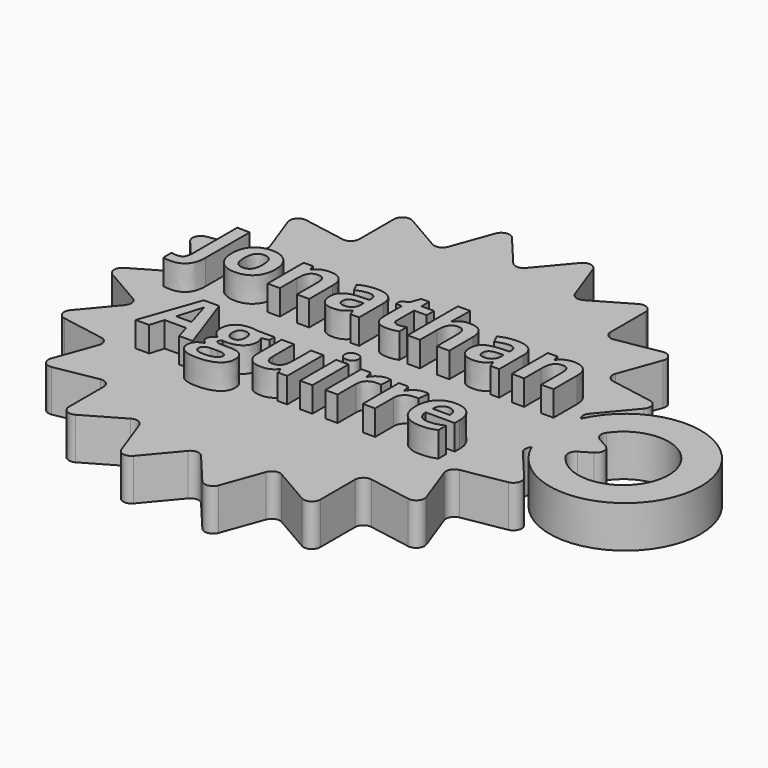
from build123d import *

# Parameters (mm, degrees)
F1_DEPTH      = 5
F2_R          = 1
F3_R          = 1
F4_R          = 9.02426598
F5_DEPTH      = 5
F7_DEPTH      = 5
F8_R          = 1
F10_DEPTH     = 4.5
F11_R         = 7.0893465871
F11_R_2       = 5.3736476411
F12_DEPTH     = 4.5
F13_TEXT_SIZE = 9.8616627859
F14_DEPTH     = 3


# Not quite as in the source:
# - a feature names something its author has since deleted; it is built from what else it names
# - Text() gives the source's letters only with a copy of the font that has no kerning and outlines rounded to 1/6400 em; it was checked with that copy


with BuildPart() as f1:
    # F0 (on Top) → F1 (new body)
    with BuildSketch(Plane.XY):
        Polygon((-69.4327632519, 10.2606042998), (-64.2233179219, 4.0522291123), (-71.2419846284, 0), (-64.2233179219, -4.0522291123), (-69.4327632519, -10.2606042998), (-61.4514299584, -11.6679287015), (-64.2233179219, -19.2836282906), (-56.2419846284, -17.8763038889), (-56.2419846284, -25.9807621135), (-49.2233179219, -21.9285330012), (-46.4514299584, -29.5442325904), (-41.2419846284, -23.3358574029), (-36.0325392983, -29.5442325904), (-33.2606513348, -21.9285330012), (-26.2419846284, -25.9807621135), (-26.2419846284, -17.8763038889), (-18.2606513348, -19.2836282906), (-21.0325392984, -11.6679287015), (-13.0512060048, -10.2606042998), (-18.2606513348, -4.0522291123), (-11.2419846284, 0), (-18.2606513348, 4.0522291123), (-13.0512060048, 10.2606042998), (-21.0325392984, 11.6679287015), (-18.2606513348, 19.2836282906), (-26.2419846284, 17.8763038889), (-26.2419846284, 25.9807621135), (-33.2606513348, 21.9285330012), (-36.0325392984, 29.5442325904), (-41.2419846284, 23.3358574029), (-46.4514299584, 29.5442325904), (-49.2233179219, 21.9285330012), (-56.2419846284, 25.9807621135), (-56.2419846284, 17.8763038889), (-64.2233179219, 19.2836282906), (-61.4514299584, 11.6679287015), align=None)
    extrude(amount=F1_DEPTH)

    # F2
    f2_edges = [f1.edges().sort_by_distance(p)[0] for p in [
        (-49.223318, -21.928533, 2.5),
        (-56.241985, -17.876304, 2.5),
        (-61.45143, -11.667929, 2.5),
        (-64.223318, -4.052229, 2.5),
        (-64.223318, 4.052229, 2.5),
        (-61.45143, 11.667929, 2.5),
        (-56.241985, 17.876304, 2.5),
        (-49.223318, 21.928533, 2.5),
        (-41.241985, 23.335857, 2.5),
        (-33.260651, 21.928533, 2.5),
        (-41.241985, -23.335857, 2.5),
        (-33.260651, -21.928533, 2.5),
        (-26.241985, -17.876304, 2.5),
        (-21.032539, -11.667929, 2.5),
        (-26.241985, 17.876304, 2.5),
        (-21.032539, 11.667929, 2.5),
        (-18.260651, 4.052229, 2.5),
        (-18.260651, -4.052229, 2.5),
    ]]
    fillet(f2_edges, radius=F2_R)

    # F3
    f3_edges = [f1.edges().sort_by_distance(p)[0] for p in [
        (-36.032539, 29.544233, 2.5),
        (-26.241985, 25.980762, 2.5),
        (-18.260651, 19.283628, 2.5),
        (-13.051206, 10.260604, 2.5),
        (-11.241985, 0, 2.5),
        (-13.051206, -10.260604, 2.5),
        (-56.241985, 25.980762, 2.5),
        (-46.45143, 29.544233, 2.5),
        (-64.223318, 19.283628, 2.5),
        (-69.432763, 10.260604, 2.5),
        (-71.241985, 0, 2.5),
        (-69.432763, -10.260604, 2.5),
        (-64.223318, -19.283628, 2.5),
        (-56.241985, -25.980762, 2.5),
        (-46.45143, -29.544233, 2.5),
        (-36.032539, -29.544233, 2.5),
        (-26.241985, -25.980762, 2.5),
        (-18.260651, -19.283628, 2.5),
    ]]
    fillet(f3_edges, radius=F3_R)

    # F4 (on Top) → F5 (join, through all)
    with BuildSketch(Plane.XY):
        with Locations((-9.2419846284, 0)):
            Circle(F4_R)
    extrude(amount=F5_DEPTH)

    # F6 (on face) → F7 (cut, through all)
    with BuildSketch(Plane.XY.offset(5)):
        with BuildLine():
            ThreePointArc((-14.3705448136, -2.1852792706), (-3.981082649, -0.0942598595), (-14.3705448136, 1.9967595517))
            Line((-14.3705448136, 1.9967595517), (-10.7515631244, 0))
            Line((-10.7515631244, 0), (-14.3705448136, -2.1852792706))
        make_face()
    extrude(amount=-F7_DEPTH, mode=Mode.SUBTRACT)

    # F8
    f8_edges = [f1.edges().sort_by_distance(p)[0] for p in [
        (-10.751563, 0, 2.5),
        (-14.370545, -2.185279, 2.5),
        (-14.370545, 1.99676, 2.5),
    ]]
    fillet(f8_edges, radius=F8_R)

    # F9 (on face) → F10 (cut)
    with BuildSketch(Plane.XY):
        with BuildLine():
            ThreePointArc((-35.3777156799, -4.6599307489), (-35.5753046169, -4.908160303), (-35.7829730175, -5.1480209603))
            Line((-35.7829730175, -5.1480209603), (-21.9766725259, -17.609254409))
            Line((-21.9766725259, -17.609254409), (-20.5904544794, -15.9396992978))
            Line((-20.5904544794, -15.9396992978), (-35.3777156799, -4.6599307489))
        make_face()
        with BuildLine():
            Line((-35.0430152336, -4.1849240607), (-22.1269458204, -12.5734481191))
            Line((-22.1269458204, -12.5734481191), (-20.8090839907, -10.2629405882))
            Line((-20.8090839907, -10.2629405882), (-34.6043804511, -3.4158988524))
            ThreePointArc((-34.6043804511, -3.4158988524), (-34.8126121734, -3.8067344742), (-35.0430152336, -4.1849240607))
        make_face()
        with BuildLine():
            ThreePointArc((-34.1823081919, -2.3833949122), (-34.2698744439, -2.6366901562), (-34.3662212872, -2.8867773708))
            Line((-34.3662212872, -2.8867773708), (-17.1305497448, -9.8744736155))
            Line((-17.1305497448, -9.8744736155), (-16.3989523541, -7.8314905025))
            Line((-16.3989523541, -7.8314905025), (-19.4509472573, -6.8787666419))
            Line((-19.4509472573, -6.8787666419), (-34.1823081919, -2.3833949122))
        make_face()
        with BuildLine():
            Line((-34.0002869576, -1.7286818538), (-18.9941076397, -5.1937600989))
            Line((-18.9941076397, -5.1937600989), (-18.54596272, -2.5718579299))
            Line((-18.54596272, -2.5718579299), (-33.8511272013, -0.8560126092))
            ThreePointArc((-33.8511272013, -0.8560126092), (-33.9131273587, -1.2944974025), (-34.0002869576, -1.7286818538))
        make_face()
        with BuildLine():
            ThreePointArc((-33.8115942061, 0.3570473634), (-33.8033972316, 0.0398847724), (-33.8083009973, -0.2773458261))
            Line((-33.8083009973, -0.2773458261), (-15.2221347635, -0.9486855723))
            Line((-15.2221347635, -0.9486855723), (-15.2333994712, 1.2213116278))
            Line((-15.2333994712, 1.2213116278), (-33.8115942061, 0.3570473634))
        make_face()
        with BuildLine():
            Line((-33.8605272028, 0.9360648973), (-18.5742046736, 2.812372041))
            Line((-18.5742046736, 2.812372041), (-19.0498295551, 5.4294287513))
            Line((-19.0498295551, 5.4294287513), (-34.0188333405, 1.807121388))
            ThreePointArc((-34.0188333405, 1.807121388), (-33.9271237992, 1.3738751607), (-33.8605272028, 0.9360648973))
        make_face()
        with BuildLine():
            ThreePointArc((-34.3965754224, 2.9605459736), (-34.2803967911, 2.6653141576), (-34.1765055688, 2.3655377184))
            Line((-34.1765055688, 2.3655377184), (-16.481610594, 8.0915279521))
            Line((-16.481610594, 8.0915279521), (-17.2343787101, 10.1268055511))
            Line((-17.2343787101, 10.1268055511), (-34.3965754224, 2.9605459736))
        make_face()
        with BuildLine():
            Line((-34.6405930582, 3.4879084069), (-20.9178834168, 10.4792906065))
            Line((-20.9178834168, 10.4792906065), (-22.2599107194, 12.7758461952))
            Line((-22.2599107194, 12.7758461952), (-35.0872710335, 4.2522898756))
            ThreePointArc((-35.0872710335, 4.2522898756), (-34.8529133175, 3.8765381033), (-34.6405930582, 3.4879084069))
        make_face()
        with BuildLine():
            ThreePointArc((-35.8367269225, 5.2069590463), (-35.6265794919, 4.9692673195), (-35.4264240963, 4.7231025025))
            Line((-35.4264240963, 4.7231025025), (-20.7570658633, 16.1557837872))
            Line((-20.7570658633, 16.1557837872), (-22.1605424433, 17.8108572693))
            Line((-22.1605424433, 17.8108572693), (-35.8367269225, 5.2069590463))
        make_face()
        with BuildLine():
            Line((-36.2463970692, 5.6190586866), (-25.742461624, 16.882252067))
            Line((-25.742461624, 16.882252067), (-27.7890230487, 18.5813080366))
            Line((-27.7890230487, 18.5813080366), (-36.927570926, 6.184569447))
            ThreePointArc((-36.927570926, 6.184569447), (-36.5788320346, 5.911633339), (-36.2463970692, 5.6190586866))
        make_face()
        with BuildLine():
            ThreePointArc((-37.958345181, 6.8253360115), (-37.6795758328, 6.6738535042), (-37.4072979585, 6.5109914192))
            Line((-37.4072979585, 6.5109914192), (-27.5328175668, 22.2714136636))
            Line((-27.5328175668, 22.2714136636), (-29.4177226221, 23.3466567405))
            Line((-29.4177226221, 23.3466567405), (-37.958345181, 6.8253360115))
        make_face()
        with BuildLine():
            Line((-38.4842555729, 7.0724675602), (-32.4660239601, 21.2489647728))
            Line((-32.4660239601, 21.2489647728), (-34.9702739951, 22.1455898979))
            Line((-34.9702739951, 22.1455898979), (-39.3177656909, 7.3708986687))
            ThreePointArc((-39.3177656909, 7.3708986687), (-38.8967086813, 7.2336983476), (-38.4842555729, 7.0724675602))
        make_face()
        with BuildLine():
            ThreePointArc((-40.5055317243, 7.6204767225), (-40.191764156, 7.5734744606), (-39.8802045331, 7.5135586787))
            Line((-39.8802045331, 7.5135586787), (-35.9916100498, 25.7007823611))
            Line((-35.9916100498, 25.7007823611), (-38.1305962124, 26.0665048489))
            Line((-38.1305962124, 26.0665048489), (-40.5055317243, 7.6204767225))
        make_face()
        with BuildLine():
            Line((-41.0842498064, 7.6728324676), (-40.2776095782, 23.0527387256))
            Line((-40.2776095782, 23.0527387256), (-42.9374987105, 23.0387867834))
            Line((-42.9374987105, 23.0387867834), (-41.9695625642, 7.668188728))
            ThreePointArc((-41.9695625642, 7.668188728), (-41.5269731258, 7.6832725775), (-41.0842498064, 7.6728324676))
        make_face()
        with BuildLine():
            ThreePointArc((-43.1710582627, 7.4964754745), (-42.8601374738, 7.5596226245), (-42.5468747909, 7.6098798733))
            Line((-42.5468747909, 7.6098798733), (-45.1131881003, 26.0302574027))
            Line((-45.1131881003, 26.0302574027), (-47.2482620709, 25.6423477718))
            Line((-47.2482620709, 25.6423477718), (-43.1710582627, 7.4964754745))
        make_face()
        with BuildLine():
            Line((-43.7327820934, 7.3477405404), (-48.235025966, 22.0760121659))
            Line((-48.235025966, 22.0760121659), (-50.7297323105, 21.1531659665))
            Line((-50.7297323105, 21.1531659665), (-44.5631157065, 7.0405820563))
            ThreePointArc((-44.5631157065, 7.0405820563), (-44.1523766576, 7.2061307415), (-43.7327820934, 7.3477405404))
        make_face()
        with BuildLine():
            ThreePointArc((-45.6334229567, 6.468288648), (-45.362850583, 6.6339687317), (-45.085668943, 6.7883372453))
            Line((-45.085668943, 6.7883372453), (-53.7973547852, 23.2200992358))
            Line((-53.7973547852, 23.2200992358), (-55.6709951327, 22.1253451128))
            Line((-55.6709951327, 22.1253451128), (-45.6334229567, 6.468288648))
        make_face()
        with BuildLine():
            Line((-46.1104003519, 6.1364026629), (-55.3784912683, 18.4365927318))
            Line((-55.3784912683, 18.4365927318), (-57.4071164218, 16.7161611466))
            Line((-57.4071164218, 16.7161611466), (-46.7856043321, 5.5637772807))
            ThreePointArc((-46.7856043321, 5.5637772807), (-46.4562568639, 5.8598231869), (-46.1104003519, 6.1364026629))
        make_face()
        with BuildLine():
            ThreePointArc((-47.5956282836, 4.6599307489), (-47.3980393467, 4.908160303), (-47.190370946, 5.1480209603))
            Line((-47.190370946, 5.1480209603), (-60.9966714376, 17.609254409))
            Line((-60.9966714376, 17.609254409), (-62.3828894841, 15.9396992978))
            Line((-62.3828894841, 15.9396992978), (-47.5956282836, 4.6599307489))
        make_face()
        with BuildLine():
            Line((-47.93032873, 4.1849240607), (-60.8463981431, 12.5734481191))
            Line((-60.8463981431, 12.5734481191), (-62.1642599729, 10.2629405882))
            Line((-62.1642599729, 10.2629405882), (-48.3689635124, 3.4158988524))
            ThreePointArc((-48.3689635124, 3.4158988524), (-48.1607317901, 3.8067344742), (-47.93032873, 4.1849240607))
        make_face()
        with BuildLine():
            ThreePointArc((-48.821003322, 2.2895164282), (-48.7202299636, 2.590355305), (-48.6071226764, 2.8867773708))
            Line((-48.6071226764, 2.8867773708), (-65.8427942188, 9.8744736155))
            Line((-65.8427942188, 9.8744736155), (-66.5743916094, 7.8314905025))
            Line((-66.5743916094, 7.8314905025), (-48.821003322, 2.2895164282))
        make_face()
        with BuildLine():
            Line((-48.973057006, 1.7286818538), (-63.9792363238, 5.1937600989))
            Line((-63.9792363238, 5.1937600989), (-64.4273812436, 2.5718579299))
            Line((-64.4273812436, 2.5718579299), (-49.1222167623, 0.8560126092))
            ThreePointArc((-49.1222167623, 0.8560126092), (-49.0602166048, 1.2944974025), (-48.973057006, 1.7286818538))
        make_face()
        Polygon((-49.1617497575, -0.3570473634), (-49.1650429663, 0.2773458261), (-67.7512092001, 0.9486855723), (-67.7399444924, -1.2213116278), align=None)
        with BuildLine():
            ThreePointArc((-48.5767685411, -2.9605459736), (-48.6929471725, -2.6653141576), (-48.7968383947, -2.3655377184))
            Line((-48.7968383947, -2.3655377184), (-66.4917333696, -8.0915279521))
            Line((-66.4917333696, -8.0915279521), (-65.7389652535, -10.1268055511))
            Line((-65.7389652535, -10.1268055511), (-48.5767685411, -2.9605459736))
        make_face()
        with BuildLine():
            Line((-49.1128167608, -0.9360648973), (-64.39913929, -2.812372041))
            Line((-64.39913929, -2.812372041), (-63.9235144085, -5.4294287513))
            Line((-63.9235144085, -5.4294287513), (-48.954510623, -1.807121388))
            ThreePointArc((-48.954510623, -1.807121388), (-49.0462201644, -1.3738751607), (-49.1128167608, -0.9360648973))
        make_face()
        with BuildLine():
            Line((-48.3327509053, -3.4879084069), (-62.0554605467, -10.4792906065))
            Line((-62.0554605467, -10.4792906065), (-60.7134332442, -12.7758461952))
            Line((-60.7134332442, -12.7758461952), (-47.88607293, -4.2522898756))
            ThreePointArc((-47.88607293, -4.2522898756), (-48.1204306461, -3.8765381033), (-48.3327509053, -3.4879084069))
        make_face()
        with BuildLine():
            ThreePointArc((-47.1366170411, -5.2069590463), (-47.3467644716, -4.9692673195), (-47.5469198672, -4.7231025025))
            Line((-47.5469198672, -4.7231025025), (-62.2162781003, -16.1557837872))
            Line((-62.2162781003, -16.1557837872), (-60.8128015203, -17.8108572693))
            Line((-60.8128015203, -17.8108572693), (-47.1366170411, -5.2069590463))
        make_face()
        with BuildLine():
            Line((-46.7269468943, -5.6190586866), (-57.2308823396, -16.882252067))
            Line((-57.2308823396, -16.882252067), (-55.1843209149, -18.5813080366))
            Line((-55.1843209149, -18.5813080366), (-46.0457730376, -6.184569447))
            ThreePointArc((-46.0457730376, -6.184569447), (-46.394511929, -5.911633339), (-46.7269468943, -5.6190586866))
        make_face()
        with BuildLine():
            ThreePointArc((-45.0149987825, -6.8253360115), (-45.2937681308, -6.6738535042), (-45.566046005, -6.5109914192))
            Line((-45.566046005, -6.5109914192), (-55.4405263967, -22.2714136636))
            Line((-55.4405263967, -22.2714136636), (-53.5556213415, -23.3466567405))
            Line((-53.5556213415, -23.3466567405), (-45.0149987825, -6.8253360115))
        make_face()
        with BuildLine():
            Line((-44.4890883907, -7.0724675602), (-50.5073200035, -21.2489647728))
            Line((-50.5073200035, -21.2489647728), (-48.0030699685, -22.1455898979))
            Line((-48.0030699685, -22.1455898979), (-43.6555782727, -7.3708986687))
            ThreePointArc((-43.6555782727, -7.3708986687), (-44.0766352823, -7.2336983476), (-44.4890883907, -7.0724675602))
        make_face()
        with BuildLine():
            ThreePointArc((-42.4678122393, -7.6204767225), (-42.7815798076, -7.5734744606), (-43.0931394305, -7.5135586787))
            Line((-43.0931394305, -7.5135586787), (-46.9817339137, -25.7007823611))
            Line((-46.9817339137, -25.7007823611), (-44.8427477512, -26.0665048489))
            Line((-44.8427477512, -26.0665048489), (-42.4678122393, -7.6204767225))
        make_face()
        with BuildLine():
            Line((-41.8890941571, -7.6728324676), (-42.6957343854, -23.0527387256))
            Line((-42.6957343854, -23.0527387256), (-40.0358452531, -23.0387867834))
            Line((-40.0358452531, -23.0387867834), (-41.0037813994, -7.668188728))
            ThreePointArc((-41.0037813994, -7.668188728), (-41.4463708377, -7.6832725775), (-41.8890941571, -7.6728324676))
        make_face()
        with BuildLine():
            ThreePointArc((-39.8022857009, -7.4964754745), (-40.1132064898, -7.5596226245), (-40.4264691727, -7.6098798733))
            Line((-40.4264691727, -7.6098798733), (-37.8601558633, -26.0302574027))
            Line((-37.8601558633, -26.0302574027), (-35.7250818926, -25.6423477718))
            Line((-35.7250818926, -25.6423477718), (-39.8022857009, -7.4964754745))
        make_face()
        with BuildLine():
            Line((-39.2405618701, -7.3477405404), (-34.7383179975, -22.0760121659))
            Line((-34.7383179975, -22.0760121659), (-32.2436116531, -21.1531659665))
            Line((-32.2436116531, -21.1531659665), (-38.4102282571, -7.0405820563))
            ThreePointArc((-38.4102282571, -7.0405820563), (-38.8209673059, -7.2061307415), (-39.2405618701, -7.3477405404))
        make_face()
        with BuildLine():
            ThreePointArc((-37.3399210068, -6.468288648), (-37.6104933805, -6.6339687317), (-37.8876750206, -6.7883372453))
            Line((-37.8876750206, -6.7883372453), (-29.1759891784, -23.2200992358))
            Line((-29.1759891784, -23.2200992358), (-27.3023488309, -22.1253451128))
            Line((-27.3023488309, -22.1253451128), (-37.3399210068, -6.468288648))
        make_face()
        with BuildLine():
            Line((-36.8629436116, -6.1364026629), (-27.5948526953, -18.4365927318))
            Line((-27.5948526953, -18.4365927318), (-25.5662275418, -16.7161611466))
            Line((-25.5662275418, -16.7161611466), (-36.1877396314, -5.5637772807))
            ThreePointArc((-36.1877396314, -5.5637772807), (-36.5170870997, -5.8598231869), (-36.8629436116, -6.1364026629))
        make_face()
    extrude(amount=F10_DEPTH, mode=Mode.SUBTRACT)

    # F11 (on face) → F12 (cut, through all)
    with BuildSketch(Plane.XY):
        with Locations((-41.4866719818, 0)):
            Circle(F11_R)
        with Locations((-41.4866719818, 0)):
            Circle(F11_R_2, mode=Mode.SUBTRACT)
    extrude(amount=F12_DEPTH, mode=Mode.SUBTRACT)

    # F13 (on face) → F14 (join)
    with BuildSketch(Plane.XY.offset(5)):
        with Locations((-63.8631587411, 2.2357032583)):
            Text('Jonathan', F13_TEXT_SIZE, font='Open Sans', font_style=FontStyle.BOLD, text_align=(TextAlign.LEFT, TextAlign.BOTTOM))
        with Locations((-58.738175862, -11.1761581306)):
            Text('Aguirre', F13_TEXT_SIZE, font='Open Sans', font_style=FontStyle.BOLD, text_align=(TextAlign.LEFT, TextAlign.BOTTOM))
    extrude(amount=F14_DEPTH)


solid = f1.part
